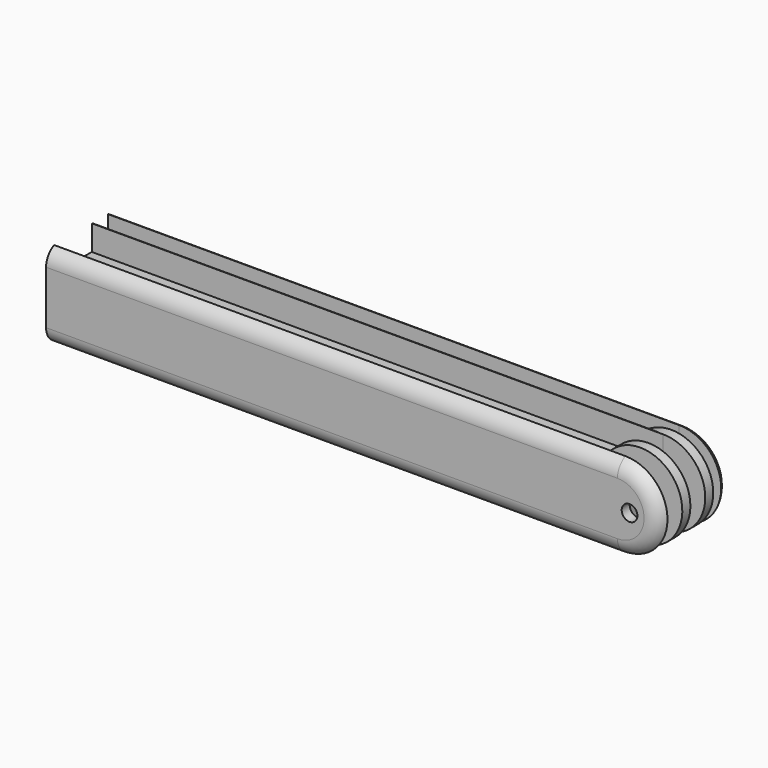
from build123d import *

# Parameters (mm, degrees)
F0_W          = 170
F0_H          = 3
F1_DEPTH      = 12.5
F0_H_2        = 14
F2_DEPTH      = 5
F3_DEPTH      = 12.5
F4_T1_DEPTH   = 192.9128784748
F4_2_T1_DEPTH = 192.9128784748
F5_W          = 2.989
F5_H          = 12.5
F5_W_2        = 1.5
F8_R          = 2.3415273596
F9_DEPTH      = 20.0010001


# Not quite as in the source:
# - a fillet or chamfer that OpenCascade refuses, or shapes differently, is made with other operations: its cross-section is extruded or revolved along the edge and cut away or added
# - a feature names something its author has since deleted; it is built from what else it names


with BuildPart() as f1:
    # F0 (on Top) → F1 (new body, symmetric)
    with BuildSketch(Plane.XY):
        with Locations((0, -11.4776883987)):
            Rectangle(F0_W, F0_H)
    extrude(amount=F1_DEPTH, both=True)

    # F4: fillet of radius 5 on 2 edges, made by hand

    # F4_s2 → F4_t1 (cut)
    with BuildSketch(Plane.YZ.offset(-96.4564392374)):
        with BuildLine():
            ThreePointArc((-12.9776883987, -7.917424305), (-12.1609885313, -10.6560370926), (-9.9776883987, -12.5))
            Line((-9.9776883987, -12.5), (-12.9776883987, -12.5))
            Line((-12.9776883987, -12.5), (-12.9776883987, -7.917424305))
        make_face()
        with BuildLine():
            ThreePointArc((-12.9776883987, 7.917424305), (-12.1609885313, 10.6560370926), (-9.9776883987, 12.5))
            Line((-9.9776883987, 12.5), (-12.9776883987, 12.5))
            Line((-12.9776883987, 12.5), (-12.9776883987, 7.917424305))
        make_face()
    extrude(amount=F4_T1_DEPTH, mode=Mode.SUBTRACT)

    # F5 (on face) → F6, piece 2 (revolve)
    with BuildSketch(Plane.YZ.offset(85)):
        with BuildLine():
            Line((-9.9885491654, 0), (-9.9885491654, 12.4952446354))
            ThreePointArc((-9.9885491654, 12.4952446354), (-12.1642325483, 10.6510753587), (-12.9776883987, 7.917424305))
            Line((-12.9776883987, 7.917424305), (-12.9776883987, 0))
            Line((-12.9776883987, 0), (-12.6429592585, 0))
            Line((-12.6429592585, 0), (-9.9885491654, 0))
        make_face()
    revolve(axis=Axis((85, -2.9776883987, 0), (0, -1, 0)))


with BuildPart() as f2:
    # F0 (on Top) → F2 (new body, symmetric)
    with BuildSketch(Plane.XY):
        with Locations((0, -2.9776883987)):
            Rectangle(F0_W, F0_H_2)
    extrude(amount=F2_DEPTH, both=True)

    # F0 (on Top) → F3 (join, symmetric)
    with BuildSketch(Plane.XY):
        with Locations((0, 5.5223116013)):
            Rectangle(F0_W, F0_H)
    extrude(amount=F3_DEPTH, both=True)

    # F4#2: fillet of radius 5 on 2 edges, made by hand

    # F4_2_s2 → F4_2_t1 (cut)
    with BuildSketch(Plane.YZ.offset(-96.4564392374)):
        with BuildLine():
            ThreePointArc((7.0223116013, -7.917424305), (6.205611734, -10.6560370926), (4.0223116013, -12.5))
            Line((4.0223116013, -12.5), (7.0223116013, -12.5))
            Line((7.0223116013, -12.5), (7.0223116013, -7.917424305))
        make_face()
        with BuildLine():
            ThreePointArc((7.0223116013, 7.917424305), (6.205611734, 10.6560370926), (4.0223116013, 12.5))
            Line((4.0223116013, 12.5), (7.0223116013, 12.5))
            Line((7.0223116013, 12.5), (7.0223116013, 7.917424305))
        make_face()
    extrude(amount=F4_2_T1_DEPTH, mode=Mode.SUBTRACT)

    # F5 (on face) → F6 (revolve)
    with BuildSketch(Plane.YZ.offset(85)):
        with Locations((5.5278116013, 6.25)):
            Rectangle(F5_W, F5_H)
    revolve(axis=Axis((85, -2.9776883987, 0), (0, -1, 0)))


with BuildPart() as f7:
    # F5 (on face) → F7 (revolve)
    with BuildSketch(Plane.YZ.offset(85)):
        with Locations((-2.2276883987, 6.25)):
            Rectangle(F5_W_2, F5_H)
        with Locations((-3.7276883987, 6.25)):
            Rectangle(F5_W_2, F5_H)
    revolve(axis=Axis((85, -2.9776883987, 0), (0, -1, 0)))


with BuildPart() as f9_tool:
    # F8 (on face) → F9 (new body, through all)
    with BuildSketch(Plane.XZ.offset(12.9776883987)):
        with Locations((88.6031761765, 0)):
            Circle(F8_R)
    extrude(amount=-F9_DEPTH)


with BuildPart() as f1_1:
    add(f1.part)

    # F9: cut by f9_tool
    add(f9_tool.part, mode=Mode.SUBTRACT)


with BuildPart() as f2_1:
    add(f2.part)

    # F9: cut by f9_tool
    add(f9_tool.part, mode=Mode.SUBTRACT)


with BuildPart() as f7_1:
    add(f7.part)

    # F9: cut by f9_tool
    add(f9_tool.part, mode=Mode.SUBTRACT)


with BuildPart() as f10_1:
    # F10: instance of F1
    add(f1_1.part.mirror(Plane.XZ))


solid = Compound([f1_1.part, f2_1.part, f7_1.part, f10_1.part])
